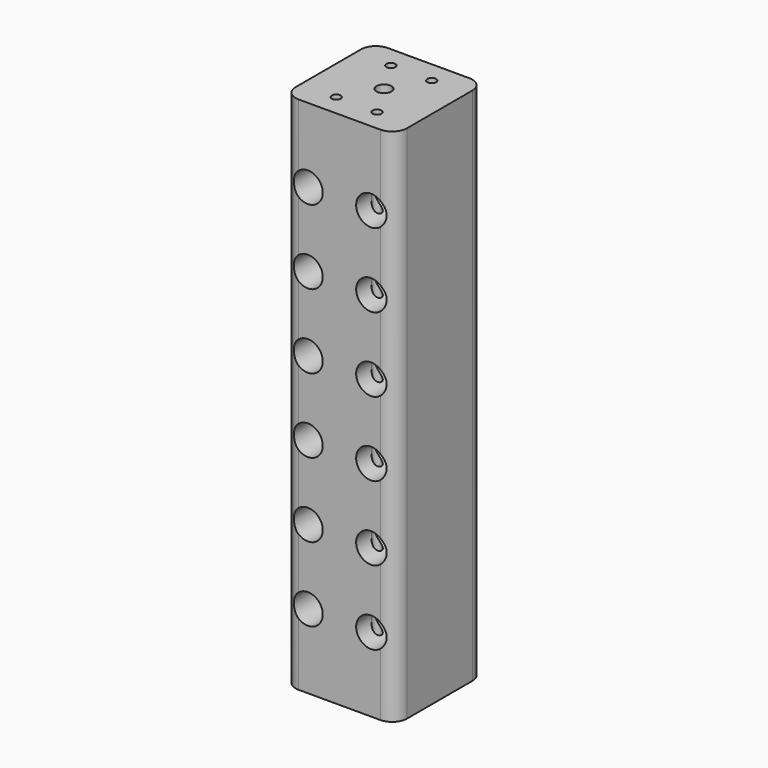
from build123d import *

# Parameters (mm, degrees)
F0_W        = 38.1
F0_H        = 38.1
F0_R        = 2.54
F1_DEPTH    = 177.8
F3_DEPTH    = 50.8
F4_T1_DEPTH = 203.2
F5_R        = 1.524
F6_DEPTH    = 177.8


# Not quite as in the source:
# - a fillet or chamfer that OpenCascade refuses, or shapes differently, is made with other operations: its cross-section is extruded or revolved along the edge and cut away or added


with BuildPart() as f1:
    # F0 (on Top) → F1 (new body)
    with BuildSketch(Plane.XY):
        Rectangle(F0_W, F0_H)
        Circle(F0_R, mode=Mode.SUBTRACT)
    extrude(amount=F1_DEPTH)

    # F2 (on face) → F3 (cut)
    with BuildSketch(Plane(origin=(0, 19.05, 0), x_dir=(-1, 0, 0), z_dir=(0, 1, 0))):
        with BuildLine():
            ThreePointArc((-15.875, 25.4), (-10.795, 20.32), (-5.715, 25.4))
            Line((-5.715, 25.4), (-15.875, 25.4))
        make_face()
        with BuildLine():
            Line((-15.875, 25.4), (-5.715, 25.4))
            ThreePointArc((-5.715, 25.4), (-10.795, 30.48), (-15.875, 25.4))
        make_face()
        with BuildLine():
            Line((15.875, 25.4), (5.715, 25.4))
            ThreePointArc((5.715, 25.4), (10.795, 20.32), (15.875, 25.4))
        make_face()
        with BuildLine():
            Line((15.875, 50.8), (5.715, 50.8))
            ThreePointArc((5.715, 50.8), (10.795, 45.72), (15.875, 50.8))
        make_face()
        with BuildLine():
            ThreePointArc((15.875, 50.8), (10.795, 55.88), (5.715, 50.8))
            Line((5.715, 50.8), (15.875, 50.8))
        make_face()
        with BuildLine():
            Line((-15.875, 50.8), (-5.715, 50.8))
            ThreePointArc((-5.715, 50.8), (-10.795, 55.88), (-15.875, 50.8))
        make_face()
        with BuildLine():
            ThreePointArc((-15.875, 50.8), (-10.795, 45.72), (-5.715, 50.8))
            Line((-5.715, 50.8), (-15.875, 50.8))
        make_face()
        with BuildLine():
            Line((-15.875, 76.2), (-5.715, 76.2))
            ThreePointArc((-5.715, 76.2), (-10.795, 81.28), (-15.875, 76.2))
        make_face()
        with BuildLine():
            Line((15.875, 76.2), (5.715, 76.2))
            ThreePointArc((5.715, 76.2), (10.795, 71.12), (15.875, 76.2))
        make_face()
        with BuildLine():
            ThreePointArc((15.875, 76.2), (10.795, 81.28), (5.715, 76.2))
            Line((5.715, 76.2), (15.875, 76.2))
        make_face()
        with BuildLine():
            Line((15.875, 101.6), (5.715, 101.6))
            ThreePointArc((5.715, 101.6), (10.795, 96.52), (15.875, 101.6))
        make_face()
        with BuildLine():
            ThreePointArc((15.875, 101.6), (10.795, 106.68), (5.715, 101.6))
            Line((5.715, 101.6), (15.875, 101.6))
        make_face()
        with BuildLine():
            ThreePointArc((-15.875, 101.6), (-10.795, 96.52), (-5.715, 101.6))
            Line((-5.715, 101.6), (-15.875, 101.6))
        make_face()
        with BuildLine():
            Line((-15.875, 101.6), (-5.715, 101.6))
            ThreePointArc((-5.715, 101.6), (-10.795, 106.68), (-15.875, 101.6))
        make_face()
        with BuildLine():
            ThreePointArc((15.875, 25.4), (10.795, 30.48), (5.715, 25.4))
            Line((5.715, 25.4), (15.875, 25.4))
        make_face()
        with BuildLine():
            Line((15.875, 127), (5.715, 127))
            ThreePointArc((5.715, 127), (10.795, 121.92), (15.875, 127))
        make_face()
        with BuildLine():
            ThreePointArc((15.875, 127), (10.795, 132.08), (5.715, 127))
            Line((5.715, 127), (15.875, 127))
        make_face()
        with BuildLine():
            ThreePointArc((-15.875, 127), (-10.795, 121.92), (-5.715, 127))
            Line((-5.715, 127), (-15.875, 127))
        make_face()
        with BuildLine():
            Line((-15.875, 127), (-5.715, 127))
            ThreePointArc((-5.715, 127), (-10.795, 132.08), (-15.875, 127))
        make_face()
        with BuildLine():
            ThreePointArc((-15.875, 152.4), (-10.795, 147.32), (-5.715, 152.4))
            Line((-5.715, 152.4), (-15.875, 152.4))
        make_face()
        with BuildLine():
            Line((-15.875, 152.4), (-5.715, 152.4))
            ThreePointArc((-5.715, 152.4), (-10.795, 157.48), (-15.875, 152.4))
        make_face()
        with BuildLine():
            Line((15.875, 152.4), (5.715, 152.4))
            ThreePointArc((5.715, 152.4), (10.795, 147.32), (15.875, 152.4))
        make_face()
        with BuildLine():
            ThreePointArc((15.875, 152.4), (10.795, 157.48), (5.715, 152.4))
            Line((5.715, 152.4), (15.875, 152.4))
        make_face()
        with BuildLine():
            ThreePointArc((-15.875, 76.2), (-10.795, 71.12), (-5.715, 76.2))
            Line((-5.715, 76.2), (-15.875, 76.2))
        make_face()
    extrude(amount=-F3_DEPTH, mode=Mode.SUBTRACT)

    # F4: fillet of radius 5.08 on 4 edges, made by hand

    # F4_s2 → F4_t1 (cut)
    with BuildSketch(Plane.XY.offset(-12.7)):
        with BuildLine():
            ThreePointArc((19.05, 13.97), (17.5621024484, 17.5621024484), (13.97, 19.05))
            Line((13.97, 19.05), (19.05, 19.05))
            Line((19.05, 19.05), (19.05, 13.97))
        make_face()
        with BuildLine():
            ThreePointArc((19.05, -13.97), (17.5621024484, -17.5621024484), (13.97, -19.05))
            Line((13.97, -19.05), (19.05, -19.05))
            Line((19.05, -19.05), (19.05, -13.97))
        make_face()
        with BuildLine():
            ThreePointArc((-13.97, -19.05), (-17.5621024484, -17.5621024484), (-19.05, -13.97))
            Line((-19.05, -13.97), (-19.05, -19.05))
            Line((-19.05, -19.05), (-13.97, -19.05))
        make_face()
        with BuildLine():
            ThreePointArc((-13.97, 19.05), (-17.5621024484, 17.5621024484), (-19.05, 13.97))
            Line((-19.05, 13.97), (-19.05, 19.05))
            Line((-19.05, 19.05), (-13.97, 19.05))
        make_face()
    extrude(amount=F4_T1_DEPTH, mode=Mode.SUBTRACT)

    # F5 (on face) → F6 (cut)
    with BuildSketch(Plane.XY.offset(177.8)):
        with Locations((-6.985, -11.684)):
            Circle(F5_R)
        with Locations((6.985, -11.684)):
            Circle(F5_R)
        with Locations((6.985, 11.684)):
            Circle(F5_R)
        with Locations((-6.985, 11.684)):
            Circle(F5_R)
    extrude(amount=-F6_DEPTH, mode=Mode.SUBTRACT)


solid = f1.part
